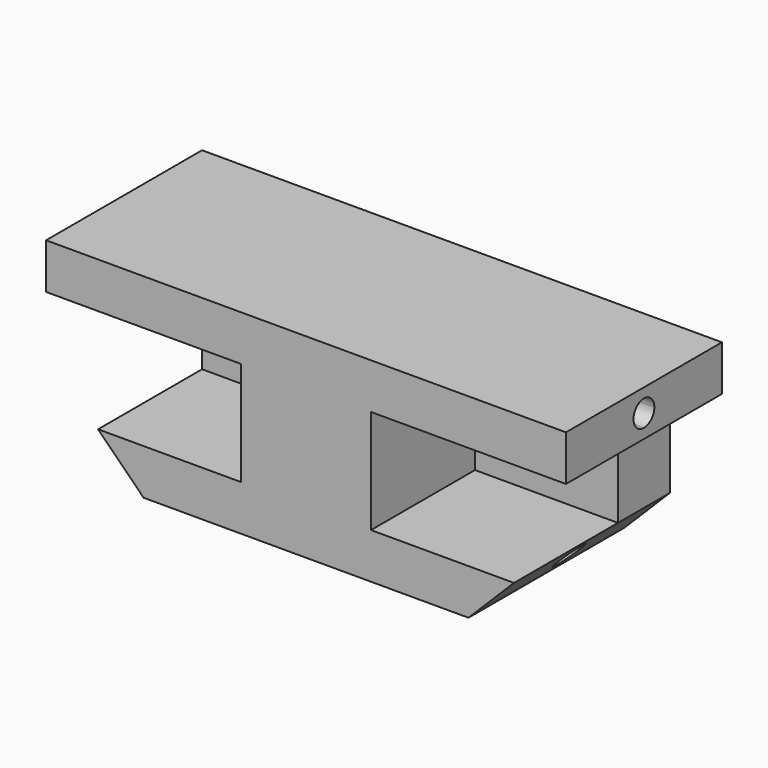
from build123d import *

# Parameters (mm, degrees)
F0_W        = 10
F0_H        = 4
F0_W_2      = 11
F1_DEPTH    = 5
F2_DEPTH    = 15
F4_DEPTH    = 40
F5_T1_DEPTH = 33.0017809158


# Not quite as in the source:
# - a fillet or chamfer that OpenCascade refuses, or shapes differently, is made with other operations: its cross-section is extruded or revolved along the edge and cut away or added


with BuildPart() as f1:
    # F0 (on Front) → F1 (new body)
    with BuildSketch(Plane.XZ):
        with Locations((0, 2)):
            Rectangle(F0_W, F0_H)
        with Locations((0, -2)):
            Rectangle(F0_W, F0_H)
        Polygon((16, -4), (5, -4), (-5, -4), (-16, -4), (-16, -7.5), (16, -7.5), align=None)
        Polygon((-5, 4), (5, 4), (16, 4), (20, 4), (20, 7.5), (-20, 7.5), (-20, 4), (-16, 4), align=None)
        with Locations((-10.5, -2)):
            Rectangle(F0_W_2, F0_H)
        with Locations((10.5, -2)):
            Rectangle(F0_W_2, F0_H)
        with Locations((10.5, 2)):
            Rectangle(F0_W_2, F0_H)
        with Locations((-10.5, 2)):
            Rectangle(F0_W_2, F0_H)
    extrude(amount=F1_DEPTH)

    # F0 (on Front) → F2 (join)
    with BuildSketch(Plane.XZ):
        Polygon((-5, 4), (5, 4), (16, 4), (20, 4), (20, 7.5), (-20, 7.5), (-20, 4), (-16, 4), align=None)
        with Locations((0, 2)):
            Rectangle(F0_W, F0_H)
        with Locations((0, -2)):
            Rectangle(F0_W, F0_H)
        Polygon((16, -4), (5, -4), (-5, -4), (-16, -4), (-16, -7.5), (16, -7.5), align=None)
    extrude(amount=F2_DEPTH)

    # F3 (on face) → F4 (cut)
    with BuildSketch(Plane.YZ.offset(20)):
        with BuildLine():
            ThreePointArc((-6.5, -5.75), (-6.7928932188, -5.0428932188), (-7.5, -4.75))
            Line((-7.5, -4.75), (-7.5, -6.75))
            ThreePointArc((-7.5, -6.75), (-6.7928932188, -6.4571067812), (-6.5, -5.75))
        make_face()
        with BuildLine():
            Line((-7.5, -6.75), (-7.5, -4.75))
            ThreePointArc((-7.5, -4.75), (-8.5, -5.75), (-7.5, -6.75))
        make_face()
        with BuildLine():
            ThreePointArc((-7.5, 6.75), (-8.5, 5.75), (-7.5, 4.75))
            Line((-7.5, 4.75), (-7.5, 6.75))
        make_face()
        with BuildLine():
            Line((-7.5, 6.75), (-7.5, 4.75))
            ThreePointArc((-7.5, 4.75), (-6.7928932188, 5.0428932188), (-6.5, 5.75))
            ThreePointArc((-6.5, 5.75), (-6.7928932188, 6.4571067812), (-7.5, 6.75))
        make_face()
    extrude(amount=-F4_DEPTH, mode=Mode.SUBTRACT)

    # F5: chamfer of 3.5 on 2 edges, made by hand

    # F5_s2 → F5_t1 (cut)
    with BuildSketch(Plane.XZ.offset(-9.0008904579)):
        Polygon((-12.5, -7.5), (-16, -4), (-16, -7.5), align=None)
        Polygon((16, -4), (12.5, -7.5), (16, -7.5), align=None)
    extrude(amount=F5_T1_DEPTH, mode=Mode.SUBTRACT)


solid = f1.part
